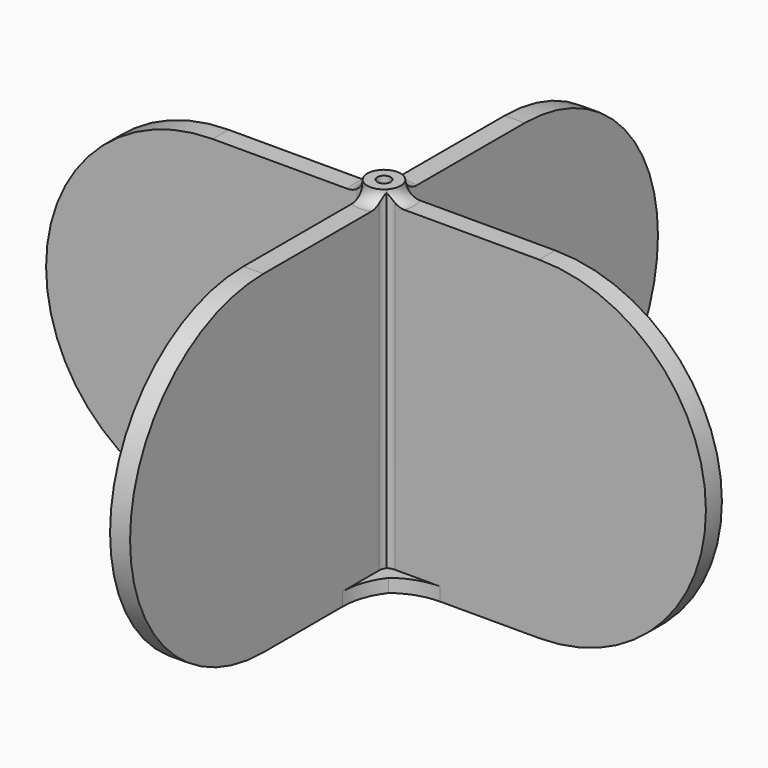
from build123d import *

# Parameters (mm, degrees)
F0_R          = 2.5
F0_R_2        = 0.5
F1_DEPTH      = 1
F2_R          = 1.25
F2_R_2        = 0.5
F3_DEPTH      = 25
F5_DEPTH      = 0.75
F5_DEPTH_BACK = 0.75
F6_COUNT      = 4
F7_T1_DEPTH   = 24
F7_T6_ANGLE   = 302.9847109955
F7_T13_ANGLE  = 302.9847109955
F7_T20_ANGLE  = 302.9847109955
F7_T27_ANGLE  = 151.4691802851
F7_T33_ANGLE  = 151.4691802851
F7_T40_DEPTH  = 25.0355339059
F7_T45_ANGLE  = 302.9847109955
F7_T53_ANGLE  = 302.9847109955
F7_T58_DEPTH  = 25.0355339059
F7_T66_ANGLE  = 302.9847109955
F7_T71_DEPTH  = 25.0355339059
F7_T79_DEPTH  = 25.0355339059
F7_T84_ANGLE  = 302.9847109955
F7_T92_ANGLE  = 302.9847109955
F7_T97_DEPTH  = 25.0355339059
F7_T105_DEPTH = 25.0355339059
F7_T110_ANGLE = 302.9847109955
F7_T118_ANGLE = 151.4691802851
F7_T123_DEPTH = 25.0355339059
F7_T131_DEPTH = 25.0355339059
F7_T136_ANGLE = 151.4691802851
F8_T1_DEPTH   = 1


# Not quite as in the source:
# - a fillet or chamfer that OpenCascade refuses, or shapes differently, is made with other operations: its cross-section is extruded or revolved along the edge and cut away or added


with BuildPart() as f1:
    # F0 (on Top) → F1 (new body)
    with BuildSketch(Plane.XY):
        Circle(F0_R)
        Circle(F0_R_2, mode=Mode.SUBTRACT)
    extrude(amount=F1_DEPTH)

    # F2 (on face) → F3 (join)
    with BuildSketch(Plane.XY.offset(1)):
        Circle(F2_R)
        Circle(F2_R_2, mode=Mode.SUBTRACT)
    extrude(amount=F3_DEPTH)

    # F4 (on Front) → F5 (join, two sides)
    with BuildSketch(Plane.XZ) as f5_sk:
        with BuildLine():
            Line((1, 25), (1, 0))
            Line((1, 0), (12.25, 0))
            ThreePointArc((12.25, 0), (24.75, 12.5), (12.25, 25))
            Line((12.25, 25), (1, 25))
        make_face()
    extrude(amount=F5_DEPTH)
    extrude(f5_sk.sketch, amount=-F5_DEPTH_BACK)

    # F6: F1 ×4 about axis
    f6_axis = Axis((0, 0, 0), (0, 0, -1))


with BuildPart() as f1_1:
    add(f1.part)
    for i in range(1, F6_COUNT):
        add(f1.part.rotate(f6_axis, i * 360 / F6_COUNT))

    # F7: fillet of radius 1 on 13 edges, made by hand

    # F7_s2 → F7_t1 (join)
    with BuildSketch(Plane.XY.offset(1)):
        with BuildLine():
            ThreePointArc((-0.7856742013, -0.9722222222), (-1.080880229, -0.8071909584), (-1.4142135624, -0.75))
            Line((-1.4142135624, -0.75), (-1.4142135624, -0.73))
            Line((-1.4142135624, -0.73), (-1, -0.73))
            Line((-1, -0.73), (-0.984, -0.738))
            ThreePointArc((-0.984, -0.738), (-0.8853286846, -0.8538694984), (-0.7731034141, -0.9566666667))
            Line((-0.7731034141, -0.9566666667), (-0.7856742013, -0.9722222222))
        make_face()
        with BuildLine():
            ThreePointArc((0.9722222222, 0.7856742013), (0.8071909584, 1.080880229), (0.75, 1.4142135624))
            Line((0.75, 1.4142135624), (0.73, 1.4142135624))
            Line((0.73, 1.4142135624), (0.73, 1))
            Line((0.73, 1), (0.738, 0.984))
            ThreePointArc((0.738, 0.984), (0.8538694984, 0.8853286846), (0.9566666667, 0.7731034141))
            Line((0.9566666667, 0.7731034141), (0.9722222222, 0.7856742013))
        make_face()
        with BuildLine():
            ThreePointArc((-0.7856742013, 0.9722222222), (-1.080880229, 0.8071909584), (-1.4142135624, 0.75))
            Line((-1.4142135624, 0.75), (-1.4142135624, 0.73))
            Line((-1.4142135624, 0.73), (-1, 0.73))
            Line((-1, 0.73), (-0.984, 0.738))
            ThreePointArc((-0.984, 0.738), (-0.8853286846, 0.8538694984), (-0.7731034141, 0.9566666667))
            Line((-0.7731034141, 0.9566666667), (-0.7856742013, 0.9722222222))
        make_face()
        with BuildLine():
            ThreePointArc((0.9722222222, -0.7856742013), (0.8071909584, -1.080880229), (0.75, -1.4142135624))
            Line((0.75, -1.4142135624), (0.73, -1.4142135624))
            Line((0.73, -1.4142135624), (0.73, -1))
            Line((0.73, -1), (0.738, -0.984))
            ThreePointArc((0.738, -0.984), (0.8538694984, -0.8853286846), (0.9566666667, -0.7731034141))
            Line((0.9566666667, -0.7731034141), (0.9722222222, -0.7856742013))
        make_face()
        with BuildLine():
            ThreePointArc((-0.9722222222, 0.7856742013), (-0.8071909584, 1.080880229), (-0.75, 1.4142135624))
            Line((-0.75, 1.4142135624), (-0.73, 1.4142135624))
            Line((-0.73, 1.4142135624), (-0.73, 1))
            Line((-0.73, 1), (-0.738, 0.984))
            ThreePointArc((-0.738, 0.984), (-0.8538694984, 0.8853286846), (-0.9566666667, 0.7731034141))
            Line((-0.9566666667, 0.7731034141), (-0.9722222222, 0.7856742013))
        make_face()
        with BuildLine():
            ThreePointArc((0.7856742013, -0.9722222222), (1.080880229, -0.8071909584), (1.4142135624, -0.75))
            Line((1.4142135624, -0.75), (1.4142135624, -0.73))
            Line((1.4142135624, -0.73), (1, -0.73))
            Line((1, -0.73), (0.984, -0.738))
            ThreePointArc((0.984, -0.738), (0.8853286846, -0.8538694984), (0.7731034141, -0.9566666667))
            Line((0.7731034141, -0.9566666667), (0.7856742013, -0.9722222222))
        make_face()
        with BuildLine():
            ThreePointArc((0.7856742013, 0.9722222222), (1.080880229, 0.8071909584), (1.4142135624, 0.75))
            Line((1.4142135624, 0.75), (1.4142135624, 0.73))
            Line((1.4142135624, 0.73), (1, 0.73))
            Line((1, 0.73), (0.984, 0.738))
            ThreePointArc((0.984, 0.738), (0.8853286846, 0.8538694984), (0.7731034141, 0.9566666667))
            Line((0.7731034141, 0.9566666667), (0.7856742013, 0.9722222222))
        make_face()
        with BuildLine():
            ThreePointArc((-0.9722222222, -0.7856742013), (-0.8071909584, -1.080880229), (-0.75, -1.4142135624))
            Line((-0.75, -1.4142135624), (-0.73, -1.4142135624))
            Line((-0.73, -1.4142135624), (-0.73, -1))
            Line((-0.73, -1), (-0.738, -0.984))
            ThreePointArc((-0.738, -0.984), (-0.8538694984, -0.8853286846), (-0.9566666667, -0.7731034141))
            Line((-0.9566666667, -0.7731034141), (-0.9722222222, -0.7856742013))
        make_face()
    extrude(amount=F7_T1_DEPTH)


with BuildPart() as f7_tool4:
    # F7_s5 → F7_t6 (revolve)
    with BuildSketch(Plane(origin=(0, 0, 0), x_dir=(0, 0, 1), z_dir=(0.4772760093, -0.8787534415, 0))):
        with BuildLine():
            ThreePointArc((26, -1.25), (25.2928932188, -1.5428932188), (25, -2.25))
            Line((25, -2.25), (24.98, -2.25))
            Line((24.98, -2.25), (24.98, -1.23))
            Line((24.98, -1.23), (26, -1.23))
            Line((26, -1.23), (26, -1.25))
        make_face()
    revolve(axis=Axis((0, 0, 25), (0, 0, 1)), revolution_arc=F7_T6_ANGLE)

    split(bisect_by=Plane.YZ.offset(-0.75), keep=Keep.BOTTOM)

    split(bisect_by=Plane.XZ.offset(-0.75), keep=Keep.TOP)

    split(bisect_by=Plane.XZ.offset(0.75), keep=Keep.BOTTOM)


with BuildPart() as f1_2:
    add(f1_1.part)

    # F7_t3: union F7_tool4
    add(f7_tool4.part)


with BuildPart() as f7_tool11:
    # F7_s12 → F7_t13 (revolve)
    with BuildSketch(Plane(origin=(0, 0, 0), x_dir=(0, 0, 1), z_dir=(0.8787534415, 0.4772760093, 0))):
        with BuildLine():
            ThreePointArc((26, -1.25), (25.2928932188, -1.5428932188), (25, -2.25))
            Line((25, -2.25), (24.98, -2.25))
            Line((24.98, -2.25), (24.98, -1.23))
            Line((24.98, -1.23), (26, -1.23))
            Line((26, -1.23), (26, -1.25))
        make_face()
    revolve(axis=Axis((0, 0, 25), (0, 0, 1)), revolution_arc=F7_T13_ANGLE)

    split(bisect_by=Plane.YZ.offset(0.75), keep=Keep.BOTTOM)

    split(bisect_by=Plane.YZ.offset(-0.75), keep=Keep.TOP)

    split(bisect_by=Plane.XZ.offset(0.75), keep=Keep.TOP)


with BuildPart() as f1_3:
    add(f1_2.part)

    # F7_t10: union F7_tool11
    add(f7_tool11.part)


with BuildPart() as f7_tool18:
    # F7_s19 → F7_t20 (revolve)
    with BuildSketch(Plane(origin=(0, 0, 0), x_dir=(0, 0, 1), z_dir=(-0.8787534415, -0.4772760093, 0))):
        with BuildLine():
            ThreePointArc((26, -1.25), (25.2928932188, -1.5428932188), (25, -2.25))
            Line((25, -2.25), (24.98, -2.25))
            Line((24.98, -2.25), (24.98, -1.23))
            Line((24.98, -1.23), (26, -1.23))
            Line((26, -1.23), (26, -1.25))
        make_face()
    revolve(axis=Axis((0, 0, 25), (0, 0, 1)), revolution_arc=F7_T20_ANGLE)

    split(bisect_by=Plane.YZ.offset(0.75), keep=Keep.BOTTOM)

    split(bisect_by=Plane.YZ.offset(-0.75), keep=Keep.TOP)

    split(bisect_by=Plane.XZ.offset(0.75), keep=Keep.BOTTOM)


with BuildPart() as f1_4:
    add(f1_3.part)

    # F7_t17: union F7_tool18
    add(f7_tool18.part)


with BuildPart() as f7_tool25:
    # F7_s26 → F7_t27 (revolve)
    with BuildSketch(Plane(origin=(0, 0, 0), x_dir=(0, 0, 1), z_dir=(-0.4776314118, -0.8785603192, 0))):
        with BuildLine():
            ThreePointArc((26, 1.25), (25.2928932188, 1.5428932188), (25, 2.25))
            Line((25, 2.25), (24.98, 2.25))
            Line((24.98, 2.25), (24.98, 1.23))
            Line((24.98, 1.23), (26, 1.23))
            Line((26, 1.23), (26, 1.25))
        make_face()
    revolve(axis=Axis((0, 0, 25), (0, 0, -1)), revolution_arc=F7_T27_ANGLE)

    split(bisect_by=Plane.YZ.offset(-0.75), keep=Keep.TOP)

    split(bisect_by=Plane.XZ.offset(-0.75), keep=Keep.TOP)


with BuildPart() as f1_5:
    add(f1_4.part)

    # F7_t24: union F7_tool25
    add(f7_tool25.part)


with BuildPart() as f7_tool31:
    # F7_s32 → F7_t33 (revolve)
    with BuildSketch(Plane.XZ):
        with BuildLine():
            ThreePointArc((1.25, 26), (1.5428932188, 25.2928932188), (2.25, 25))
            Line((2.25, 25), (2.25, 24.98))
            Line((2.25, 24.98), (1.23, 24.98))
            Line((1.23, 24.98), (1.23, 26))
            Line((1.23, 26), (1.25, 26))
        make_face()
    revolve(axis=Axis((0, 0, 25), (0, 0, -1)), revolution_arc=F7_T33_ANGLE)

    split(bisect_by=Plane.XZ.offset(0.75), keep=Keep.BOTTOM)

    split(bisect_by=Plane.YZ.offset(0.75), keep=Keep.TOP)


with BuildPart() as f1_6:
    add(f1_5.part)

    # F7_t30: union F7_tool31
    add(f7_tool31.part)


with BuildPart() as f7_tool38:
    # F7_s39 → F7_t40 (new body)
    with BuildSketch(Plane.XY.offset(26.0355339059)):
        with BuildLine():
            ThreePointArc((-0.7856742013, -0.9722222222), (-1.080880229, -0.8071909584), (-1.4142135624, -0.75))
            Line((-1.4142135624, -0.75), (-1.4142135624, -0.73))
            Line((-1.4142135624, -0.73), (-1, -0.73))
            Line((-1, -0.73), (-0.984, -0.738))
            ThreePointArc((-0.984, -0.738), (-0.8853286846, -0.8538694984), (-0.7731034141, -0.9566666667))
            Line((-0.7731034141, -0.9566666667), (-0.7856742013, -0.9722222222))
        make_face()
    extrude(amount=-F7_T40_DEPTH)

    split(bisect_by=Plane.XY.offset(26), keep=Keep.BOTTOM)

    split(bisect_by=Plane.XY.offset(25), keep=Keep.TOP)


with BuildPart() as f7_tool43:
    # F7_s44 → F7_t45 (revolve)
    with BuildSketch(Plane(origin=(0, 0, 0), x_dir=(0, 0, 1), z_dir=(0.4772760093, -0.8787534415, 0))):
        with BuildLine():
            ThreePointArc((26, -1.25), (25.2928932188, -1.5428932188), (25, -2.25))
            Line((25, -2.25), (24.98, -2.25))
            Line((24.98, -2.25), (24.98, -1.23))
            Line((24.98, -1.23), (26, -1.23))
            Line((26, -1.23), (26, -1.25))
        make_face()
    revolve(axis=Axis((0, 0, 25), (0, 0, 1)), revolution_arc=F7_T45_ANGLE)

    split(bisect_by=Plane.YZ.offset(-0.75), keep=Keep.BOTTOM)

    split(bisect_by=Plane.XZ.offset(0.75), keep=Keep.TOP)


with BuildPart() as f7_tool38_1:
    add(f7_tool38.part)

    # F7_t48: intersect F7_tool43
    add(f7_tool43.part, mode=Mode.INTERSECT)


with BuildPart() as f1_7:
    add(f1_6.part)

    # F7_t36: union F7_tool38
    add(f7_tool38_1.part)


with BuildPart() as f7_tool51:
    # F7_s52 → F7_t53 (revolve)
    with BuildSketch(Plane(origin=(0, 0, 0), x_dir=(0, 0, 1), z_dir=(-0.8787534415, -0.4772760093, 0))):
        with BuildLine():
            ThreePointArc((26, -1.25), (25.2928932188, -1.5428932188), (25, -2.25))
            Line((25, -2.25), (24.98, -2.25))
            Line((24.98, -2.25), (24.98, -1.23))
            Line((24.98, -1.23), (26, -1.23))
            Line((26, -1.23), (26, -1.25))
        make_face()
    revolve(axis=Axis((0, 0, 25), (0, 0, 1)), revolution_arc=F7_T53_ANGLE)

    split(bisect_by=Plane.YZ.offset(0.75), keep=Keep.TOP)

    split(bisect_by=Plane.XZ.offset(-0.75), keep=Keep.BOTTOM)


with BuildPart() as f7_tool56:
    # F7_s57 → F7_t58 (new body)
    with BuildSketch(Plane.XY.offset(26.0355339059)):
        with BuildLine():
            ThreePointArc((0.9722222222, 0.7856742013), (0.8071909584, 1.080880229), (0.75, 1.4142135624))
            Line((0.75, 1.4142135624), (0.73, 1.4142135624))
            Line((0.73, 1.4142135624), (0.73, 1))
            Line((0.73, 1), (0.738, 0.984))
            ThreePointArc((0.738, 0.984), (0.8538694984, 0.8853286846), (0.9566666667, 0.7731034141))
            Line((0.9566666667, 0.7731034141), (0.9722222222, 0.7856742013))
        make_face()
    extrude(amount=-F7_T58_DEPTH)

    split(bisect_by=Plane.XY.offset(26), keep=Keep.BOTTOM)

    split(bisect_by=Plane.XY.offset(25), keep=Keep.TOP)


with BuildPart() as f7_tool51_1:
    add(f7_tool51.part)

    # F7_t61: intersect F7_tool56
    add(f7_tool56.part, mode=Mode.INTERSECT)


with BuildPart() as f1_8:
    add(f1_7.part)

    # F7_t49: union F7_tool51
    add(f7_tool51_1.part)


with BuildPart() as f7_tool64:
    # F7_s65 → F7_t66 (revolve)
    with BuildSketch(Plane(origin=(0, 0, 0), x_dir=(0, 0, 1), z_dir=(0.4772760093, -0.8787534415, 0))):
        with BuildLine():
            ThreePointArc((26, -1.25), (25.2928932188, -1.5428932188), (25, -2.25))
            Line((25, -2.25), (24.98, -2.25))
            Line((24.98, -2.25), (24.98, -1.23))
            Line((24.98, -1.23), (26, -1.23))
            Line((26, -1.23), (26, -1.25))
        make_face()
    revolve(axis=Axis((0, 0, 25), (0, 0, 1)), revolution_arc=F7_T66_ANGLE)

    split(bisect_by=Plane.YZ.offset(-0.75), keep=Keep.BOTTOM)

    split(bisect_by=Plane.XZ.offset(-0.75), keep=Keep.BOTTOM)


with BuildPart() as f7_tool69:
    # F7_s70 → F7_t71 (new body)
    with BuildSketch(Plane.XY.offset(26.0355339059)):
        with BuildLine():
            ThreePointArc((-0.7856742013, 0.9722222222), (-1.080880229, 0.8071909584), (-1.4142135624, 0.75))
            Line((-1.4142135624, 0.75), (-1.4142135624, 0.73))
            Line((-1.4142135624, 0.73), (-1, 0.73))
            Line((-1, 0.73), (-0.984, 0.738))
            ThreePointArc((-0.984, 0.738), (-0.8853286846, 0.8538694984), (-0.7731034141, 0.9566666667))
            Line((-0.7731034141, 0.9566666667), (-0.7856742013, 0.9722222222))
        make_face()
    extrude(amount=-F7_T71_DEPTH)

    split(bisect_by=Plane.XY.offset(26), keep=Keep.BOTTOM)

    split(bisect_by=Plane.XY.offset(25), keep=Keep.TOP)


with BuildPart() as f7_tool64_1:
    add(f7_tool64.part)

    # F7_t74: intersect F7_tool69
    add(f7_tool69.part, mode=Mode.INTERSECT)


with BuildPart() as f1_9:
    add(f1_8.part)

    # F7_t62: union F7_tool64
    add(f7_tool64_1.part)


with BuildPart() as f7_tool77:
    # F7_s78 → F7_t79 (new body)
    with BuildSketch(Plane.XY.offset(26.0355339059)):
        with BuildLine():
            ThreePointArc((0.9722222222, -0.7856742013), (0.8071909584, -1.080880229), (0.75, -1.4142135624))
            Line((0.75, -1.4142135624), (0.73, -1.4142135624))
            Line((0.73, -1.4142135624), (0.73, -1))
            Line((0.73, -1), (0.738, -0.984))
            ThreePointArc((0.738, -0.984), (0.8538694984, -0.8853286846), (0.9566666667, -0.7731034141))
            Line((0.9566666667, -0.7731034141), (0.9722222222, -0.7856742013))
        make_face()
    extrude(amount=-F7_T79_DEPTH)

    split(bisect_by=Plane.XY.offset(26), keep=Keep.BOTTOM)

    split(bisect_by=Plane.XY.offset(25), keep=Keep.TOP)


with BuildPart() as f7_tool82:
    # F7_s83 → F7_t84 (revolve)
    with BuildSketch(Plane(origin=(0, 0, 0), x_dir=(0, 0, 1), z_dir=(0.8787534415, 0.4772760093, 0))):
        with BuildLine():
            ThreePointArc((26, -1.25), (25.2928932188, -1.5428932188), (25, -2.25))
            Line((25, -2.25), (24.98, -2.25))
            Line((24.98, -2.25), (24.98, -1.23))
            Line((24.98, -1.23), (26, -1.23))
            Line((26, -1.23), (26, -1.25))
        make_face()
    revolve(axis=Axis((0, 0, 25), (0, 0, 1)), revolution_arc=F7_T84_ANGLE)

    split(bisect_by=Plane.YZ.offset(0.75), keep=Keep.TOP)

    split(bisect_by=Plane.XZ.offset(0.75), keep=Keep.TOP)


with BuildPart() as f7_tool77_1:
    add(f7_tool77.part)

    # F7_t87: intersect F7_tool82
    add(f7_tool82.part, mode=Mode.INTERSECT)


with BuildPart() as f1_10:
    add(f1_9.part)

    # F7_t75: union F7_tool77
    add(f7_tool77_1.part)


with BuildPart() as f7_tool90:
    # F7_s91 → F7_t92 (revolve)
    with BuildSketch(Plane(origin=(0, 0, 0), x_dir=(0, 0, 1), z_dir=(0.8787534415, 0.4772760093, 0))):
        with BuildLine():
            ThreePointArc((26, -1.25), (25.2928932188, -1.5428932188), (25, -2.25))
            Line((25, -2.25), (24.98, -2.25))
            Line((24.98, -2.25), (24.98, -1.23))
            Line((24.98, -1.23), (26, -1.23))
            Line((26, -1.23), (26, -1.25))
        make_face()
    revolve(axis=Axis((0, 0, 25), (0, 0, 1)), revolution_arc=F7_T92_ANGLE)

    split(bisect_by=Plane.YZ.offset(-0.75), keep=Keep.BOTTOM)

    split(bisect_by=Plane.XZ.offset(0.75), keep=Keep.TOP)


with BuildPart() as f7_tool95:
    # F7_s96 → F7_t97 (new body)
    with BuildSketch(Plane.XY.offset(26.0355339059)):
        with BuildLine():
            ThreePointArc((-0.9722222222, -0.7856742013), (-0.8071909584, -1.080880229), (-0.75, -1.4142135624))
            Line((-0.75, -1.4142135624), (-0.73, -1.4142135624))
            Line((-0.73, -1.4142135624), (-0.73, -1))
            Line((-0.73, -1), (-0.738, -0.984))
            ThreePointArc((-0.738, -0.984), (-0.8538694984, -0.8853286846), (-0.9566666667, -0.7731034141))
            Line((-0.9566666667, -0.7731034141), (-0.9722222222, -0.7856742013))
        make_face()
    extrude(amount=-F7_T97_DEPTH)

    split(bisect_by=Plane.XY.offset(26), keep=Keep.BOTTOM)

    split(bisect_by=Plane.XY.offset(25), keep=Keep.TOP)


with BuildPart() as f7_tool90_1:
    add(f7_tool90.part)

    # F7_t100: intersect F7_tool95
    add(f7_tool95.part, mode=Mode.INTERSECT)


with BuildPart() as f1_11:
    add(f1_10.part)

    # F7_t88: union F7_tool90
    add(f7_tool90_1.part)


with BuildPart() as f7_tool103:
    # F7_s104 → F7_t105 (new body)
    with BuildSketch(Plane.XY.offset(26.0355339059)):
        with BuildLine():
            ThreePointArc((-0.9722222222, 0.7856742013), (-0.8071909584, 1.080880229), (-0.75, 1.4142135624))
            Line((-0.75, 1.4142135624), (-0.73, 1.4142135624))
            Line((-0.73, 1.4142135624), (-0.73, 1))
            Line((-0.73, 1), (-0.738, 0.984))
            ThreePointArc((-0.738, 0.984), (-0.8538694984, 0.8853286846), (-0.9566666667, 0.7731034141))
            Line((-0.9566666667, 0.7731034141), (-0.9722222222, 0.7856742013))
        make_face()
    extrude(amount=-F7_T105_DEPTH)

    split(bisect_by=Plane.XY.offset(26), keep=Keep.BOTTOM)

    split(bisect_by=Plane.XY.offset(25), keep=Keep.TOP)


with BuildPart() as f7_tool108:
    # F7_s109 → F7_t110 (revolve)
    with BuildSketch(Plane(origin=(0, 0, 0), x_dir=(0, 0, 1), z_dir=(-0.8787534415, -0.4772760093, 0))):
        with BuildLine():
            ThreePointArc((26, -1.25), (25.2928932188, -1.5428932188), (25, -2.25))
            Line((25, -2.25), (24.98, -2.25))
            Line((24.98, -2.25), (24.98, -1.23))
            Line((24.98, -1.23), (26, -1.23))
            Line((26, -1.23), (26, -1.25))
        make_face()
    revolve(axis=Axis((0, 0, 25), (0, 0, 1)), revolution_arc=F7_T110_ANGLE)

    split(bisect_by=Plane.YZ.offset(-0.75), keep=Keep.BOTTOM)

    split(bisect_by=Plane.XZ.offset(-0.75), keep=Keep.BOTTOM)


with BuildPart() as f7_tool103_1:
    add(f7_tool103.part)

    # F7_t113: intersect F7_tool108
    add(f7_tool108.part, mode=Mode.INTERSECT)


with BuildPart() as f1_12:
    add(f1_11.part)

    # F7_t101: union F7_tool103
    add(f7_tool103_1.part)


with BuildPart() as f7_tool116:
    # F7_s117 → F7_t118 (revolve)
    with BuildSketch(Plane.XZ):
        with BuildLine():
            ThreePointArc((1.25, 26), (1.5428932188, 25.2928932188), (2.25, 25))
            Line((2.25, 25), (2.25, 24.98))
            Line((2.25, 24.98), (1.23, 24.98))
            Line((1.23, 24.98), (1.23, 26))
            Line((1.23, 26), (1.25, 26))
        make_face()
    revolve(axis=Axis((0, 0, 25), (0, 0, -1)), revolution_arc=F7_T118_ANGLE)

    split(bisect_by=Plane.XZ.offset(0.75), keep=Keep.TOP)

    split(bisect_by=Plane.YZ.offset(0.75), keep=Keep.TOP)


with BuildPart() as f7_tool121:
    # F7_s122 → F7_t123 (new body)
    with BuildSketch(Plane.XY.offset(26.0355339059)):
        with BuildLine():
            ThreePointArc((0.7856742013, -0.9722222222), (1.080880229, -0.8071909584), (1.4142135624, -0.75))
            Line((1.4142135624, -0.75), (1.4142135624, -0.73))
            Line((1.4142135624, -0.73), (1, -0.73))
            Line((1, -0.73), (0.984, -0.738))
            ThreePointArc((0.984, -0.738), (0.8853286846, -0.8538694984), (0.7731034141, -0.9566666667))
            Line((0.7731034141, -0.9566666667), (0.7856742013, -0.9722222222))
        make_face()
    extrude(amount=-F7_T123_DEPTH)

    split(bisect_by=Plane.XY.offset(26), keep=Keep.BOTTOM)

    split(bisect_by=Plane.XY.offset(25), keep=Keep.TOP)


with BuildPart() as f7_tool116_1:
    add(f7_tool116.part)

    # F7_t126: intersect F7_tool121
    add(f7_tool121.part, mode=Mode.INTERSECT)


with BuildPart() as f1_13:
    add(f1_12.part)

    # F7_t114: union F7_tool116
    add(f7_tool116_1.part)


with BuildPart() as f7_tool129:
    # F7_s130 → F7_t131 (new body)
    with BuildSketch(Plane.XY.offset(26.0355339059)):
        with BuildLine():
            ThreePointArc((0.7856742013, 0.9722222222), (1.080880229, 0.8071909584), (1.4142135624, 0.75))
            Line((1.4142135624, 0.75), (1.4142135624, 0.73))
            Line((1.4142135624, 0.73), (1, 0.73))
            Line((1, 0.73), (0.984, 0.738))
            ThreePointArc((0.984, 0.738), (0.8853286846, 0.8538694984), (0.7731034141, 0.9566666667))
            Line((0.7731034141, 0.9566666667), (0.7856742013, 0.9722222222))
        make_face()
    extrude(amount=-F7_T131_DEPTH)

    split(bisect_by=Plane.XY.offset(26), keep=Keep.BOTTOM)

    split(bisect_by=Plane.XY.offset(25), keep=Keep.TOP)


with BuildPart() as f7_tool134:
    # F7_s135 → F7_t136 (revolve)
    with BuildSketch(Plane(origin=(0, 0, 0), x_dir=(0, 0, 1), z_dir=(-0.4776314118, -0.8785603192, 0))):
        with BuildLine():
            ThreePointArc((26, 1.25), (25.2928932188, 1.5428932188), (25, 2.25))
            Line((25, 2.25), (24.98, 2.25))
            Line((24.98, 2.25), (24.98, 1.23))
            Line((24.98, 1.23), (26, 1.23))
            Line((26, 1.23), (26, 1.25))
        make_face()
    revolve(axis=Axis((0, 0, 25), (0, 0, -1)), revolution_arc=F7_T136_ANGLE)

    split(bisect_by=Plane.YZ.offset(0.75), keep=Keep.TOP)

    split(bisect_by=Plane.XZ.offset(-0.75), keep=Keep.BOTTOM)


with BuildPart() as f7_tool129_1:
    add(f7_tool129.part)

    # F7_t139: intersect F7_tool134
    add(f7_tool134.part, mode=Mode.INTERSECT)


with BuildPart() as f1_14:
    add(f1_13.part)

    # F7_t127: union F7_tool129
    add(f7_tool129_1.part)

    # F8: fillet of radius 5 on 8 edges, made by hand

    # F8_s2 → F8_t1 (join)
    with BuildSketch(Plane.XY):
        with BuildLine():
            ThreePointArc((-1.9166666667, -1.605113357), (-1.0507092734, -3.1075149434), (-0.75, -4.8153400711))
            Line((-0.75, -4.8153400711), (-0.75, -2.3848480035))
            ThreePointArc((-0.75, -2.3848480035), (-1.3891631681, -2.0785152615), (-1.9166666667, -1.605113357))
        make_face()
        with BuildLine():
            ThreePointArc((4.8153400711, 0.75), (3.1075149434, 1.0507092734), (1.605113357, 1.9166666667))
            ThreePointArc((1.605113357, 1.9166666667), (2.0785152615, 1.3891631681), (2.3848480035, 0.75))
            Line((2.3848480035, 0.75), (4.8153400711, 0.75))
        make_face()
        with BuildLine():
            ThreePointArc((0.75, -4.8153400711), (1.0507092734, -3.1075149434), (1.9166666667, -1.605113357))
            ThreePointArc((1.9166666667, -1.605113357), (1.3891631681, -2.0785152615), (0.75, -2.3848480035))
            Line((0.75, -2.3848480035), (0.75, -4.8153400711))
        make_face()
        with BuildLine():
            ThreePointArc((-1.605113357, 1.9166666667), (-3.1075149434, 1.0507092734), (-4.8153400711, 0.75))
            Line((-4.8153400711, 0.75), (-2.3848480035, 0.75))
            ThreePointArc((-2.3848480035, 0.75), (-2.0785152615, 1.3891631681), (-1.605113357, 1.9166666667))
        make_face()
        with BuildLine():
            ThreePointArc((-1.605113357, -1.9166666667), (-3.1075149434, -1.0507092734), (-4.8153400711, -0.75))
            Line((-4.8153400711, -0.75), (-2.3848480035, -0.75))
            ThreePointArc((-2.3848480035, -0.75), (-2.0785152615, -1.3891631681), (-1.605113357, -1.9166666667))
        make_face()
        with BuildLine():
            ThreePointArc((1.9166666667, 1.605113357), (1.0507092734, 3.1075149434), (0.75, 4.8153400711))
            Line((0.75, 4.8153400711), (0.75, 2.3848480035))
            ThreePointArc((0.75, 2.3848480035), (1.3891631681, 2.0785152615), (1.9166666667, 1.605113357))
        make_face()
        with BuildLine():
            ThreePointArc((-0.75, 4.8153400711), (-1.0507092734, 3.1075149434), (-1.9166666667, 1.605113357))
            ThreePointArc((-1.9166666667, 1.605113357), (-1.3891631681, 2.0785152615), (-0.75, 2.3848480035))
            Line((-0.75, 2.3848480035), (-0.75, 4.8153400711))
        make_face()
        with BuildLine():
            ThreePointArc((1.605113357, -1.9166666667), (3.1075149434, -1.0507092734), (4.8153400711, -0.75))
            Line((4.8153400711, -0.75), (2.3848480035, -0.75))
            ThreePointArc((2.3848480035, -0.75), (2.0785152615, -1.3891631681), (1.605113357, -1.9166666667))
        make_face()
    extrude(amount=F8_T1_DEPTH)


solid = f1_14.part
